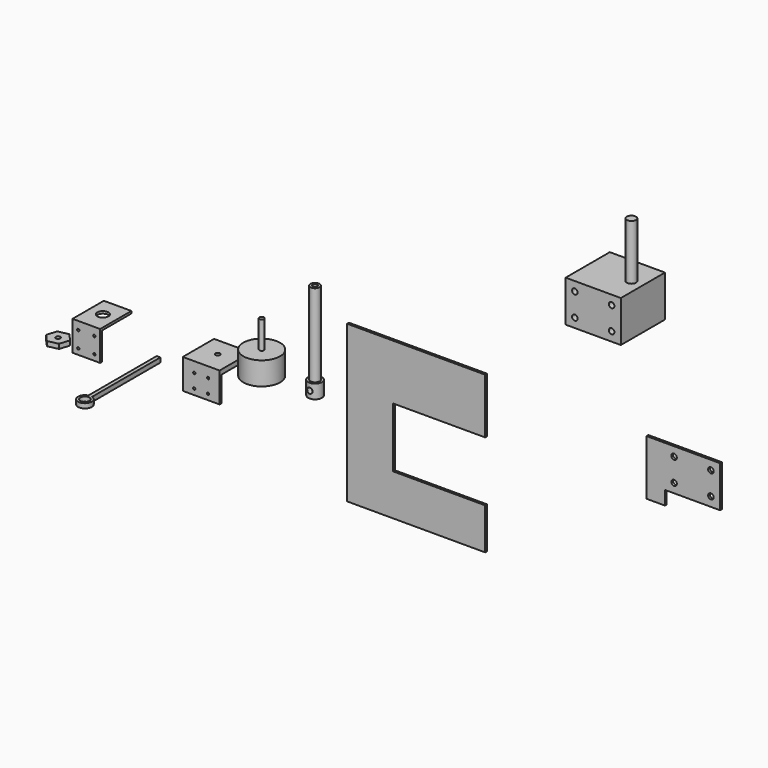
from build123d import *

# Parameters (mm, degrees)
F0_R      = 2.5
F1_DEPTH  = 15
F2_R      = 5
F2_R_2    = 2.5
F3_DEPTH  = 90
F5_R      = 3
F6_DEPTH  = 15.001
F0_R_2    = 20
F7_DEPTH  = 25
F8_R      = 2.5
F9_DEPTH  = 30
F0_W      = 40
F0_H      = 40
F10_DEPTH = 5
F11_W     = 40
F11_H     = 2.5
F12_DEPTH = 32.5
F14_DEPTH = 2.5
F0_W_2    = 30
F0_R_3    = 6
F16_DEPTH = 2.5
F17_W     = 30
F17_H     = 2.5
F18_DEPTH = 32.5
F19_DEPTH = 5
F20_R     = 1.25
F21_DEPTH = 2.5
F22_R     = 1.25
F23_DEPTH = 2.5
F13_W     = 60
F13_H     = 45
F13_R     = 3
F24_DEPTH = 60
F25_R     = 5
F26_DEPTH = 60
F27_DEPTH = 2.5
F28_R     = 3
F29_DEPTH = 25
F0_R_4    = 5
F30_DEPTH = 5


with BuildPart() as f1:
    # F0 (on Top) → F1 (new body)
    with BuildSketch(Plane.XY):
        with BuildLine():
            ThreePointArc((0, 7.5), (-5.3033008589, -5.3033008589), (7.5, 0))
            ThreePointArc((7.5, 0), (5.3033008589, 5.3033008589), (0, 7.5))
        make_face()
        Circle(F0_R, mode=Mode.SUBTRACT)
    extrude(amount=F1_DEPTH)

    # F2 (on face) → F3 (join)
    with BuildSketch(Plane.XY.offset(15)):
        Circle(F2_R)
        Circle(F2_R_2, mode=Mode.SUBTRACT)
    extrude(amount=F3_DEPTH)

    # F5 (on face) → F6 (cut, through all)
    with BuildSketch(Plane.XZ.offset(-7.5)):
        with Locations((0, 7.5)):
            Circle(F5_R)
    extrude(amount=F6_DEPTH, mode=Mode.SUBTRACT)


with BuildPart() as f7:
    # F0 (on Top) → F7 (new body)
    with BuildSketch(Plane.XY):
        with Locations((-57.9745993018, 0)):
            Circle(F0_R_2)
    extrude(amount=F7_DEPTH)

    # F8 (on face) → F9 (join)
    with BuildSketch(Plane.XY.offset(25)):
        with Locations((-57.9745993018, 0)):
            Circle(F8_R)
    extrude(amount=F9_DEPTH)


with BuildPart() as f10:
    # F0 (on Top) → F10 (new body)
    with BuildSketch(Plane.XY):
        with Locations((-105.7388707995, 0)):
            Rectangle(F0_W, F0_H)
        with Locations((-105.7388707995, 0)):
            Circle(F0_R, mode=Mode.SUBTRACT)
    extrude(amount=F10_DEPTH)

    # F11 (on face) → F12 (join)
    with BuildSketch(Plane.XY.offset(5)):
        with Locations((-105.7388707995, -21.25)):
            Rectangle(F11_W, F11_H)
    extrude(amount=-F12_DEPTH)

    # F20 (on face) → F21 (cut, through all)
    with BuildSketch(Plane(origin=(0, -20, 0), x_dir=(-1, 0, 0), z_dir=(0, 1, 0))):
        with Locations((98.2388707995, -6.25)):
            Circle(F20_R)
        with Locations((113.2388707995, -6.25)):
            Circle(F20_R)
        with Locations((113.2388707995, -21.25)):
            Circle(F20_R)
        with Locations((98.2388707995, -21.25)):
            Circle(F20_R)
    extrude(amount=-F21_DEPTH, mode=Mode.SUBTRACT)


with BuildPart() as f14:
    # F13 (on Front) → F14 (new body)
    with BuildSketch(Plane.XZ):
        Polygon((186.8768878281, 81.5050628316), (36.8768878281, 81.5050628316), (36.8768878281, -88.4949371684), (186.8768878281, -88.4949371684), (186.8768878281, -43.4949371684), (86.8768878281, -43.4949371684), (86.8768878281, 21.5050628316), (186.8768878281, 21.5050628316), align=None)
    extrude(amount=F14_DEPTH)


with BuildPart() as f16:
    # F0 (on Top) → F16 (new body)
    with BuildSketch(Plane.XY):
        with Locations((-230.5557584763, 0)):
            Rectangle(F0_W_2, F0_H)
        with Locations((-230.5557584763, 0)):
            Circle(F0_R_3, mode=Mode.SUBTRACT)
    extrude(amount=F16_DEPTH)

    # F17 (on face) → F18 (join)
    with BuildSketch(Plane.XY.offset(2.5)):
        with Locations((-230.5557584763, -21.25)):
            Rectangle(F17_W, F17_H)
    extrude(amount=-F18_DEPTH)

    # F22 (on face) → F23 (cut, through all)
    with BuildSketch(Plane(origin=(0, -20, 0), x_dir=(-1, 0, 0), z_dir=(0, 1, 0))):
        with Locations((221.8057584763, -6.25)):
            Circle(F22_R)
        with Locations((221.8057584763, -23.75)):
            Circle(F22_R)
        with Locations((239.3057584763, -23.75)):
            Circle(F22_R)
        with Locations((239.3057584763, -6.25)):
            Circle(F22_R)
    extrude(amount=-F23_DEPTH, mode=Mode.SUBTRACT)


with BuildPart() as f19:
    # F0 (on Top) → F19 (new body)
    with BuildSketch(Plane.XY):
        Polygon((-222.9001823011, -69.3075905842), (-219.3971571383, -58.4452201324), (-227.0527333135, -49.9803261255), (-238.2113346515, -52.3778025704), (-241.7143598142, -63.2401730222), (-234.058783639, -71.7050670291), align=None)
        with Locations((-230.5557584763, -60.8426965773)):
            Circle(F0_R, mode=Mode.SUBTRACT)
    extrude(amount=F19_DEPTH)


with BuildPart() as f24:
    # F13 (on Front) → F24 (new body)
    with BuildSketch(Plane.XZ):
        with Locations((302.3541259766, 178.6684757471)):
            Rectangle(F13_W, F13_H)
        with Locations((282.3541259766, 166.1684757471)):
            Circle(F13_R, mode=Mode.SUBTRACT)
        with Locations((282.3541259766, 191.1684757471)):
            Circle(F13_R, mode=Mode.SUBTRACT)
        with Locations((322.3541259766, 166.1684757471)):
            Circle(F13_R, mode=Mode.SUBTRACT)
        with Locations((322.3541259766, 191.1684757471)):
            Circle(F13_R, mode=Mode.SUBTRACT)
    extrude(amount=-F24_DEPTH)

    # F25 (on face) → F26 (join)
    with BuildSketch(Plane.XY.offset(201.1684757471)):
        with Locations((319.8541259766, 30)):
            Circle(F25_R)
    extrude(amount=F26_DEPTH)


with BuildPart() as f27:
    # F15 (on face) → F27 (new body)
    with BuildSketch(Plane.XZ.offset(2.5)):
        Polygon((444.2156124115, 81.5050628316), (364.2156124115, 81.5050628316), (364.2156124115, 21.5050628316), (384.2156124115, 21.5050628316), (384.2156124115, 36.5050628316), (444.2156124115, 36.5050628316), align=None)
    extrude(amount=F27_DEPTH)

    # F28 (on face) → F29 (cut)
    with BuildSketch(Plane.XZ.offset(5)):
        with Locations((394.2156124115, 71.5050628316)):
            Circle(F28_R)
        with Locations((394.2156124115, 46.5050628316)):
            Circle(F28_R)
        with Locations((434.2156124115, 71.5050628316)):
            Circle(F28_R)
        with Locations((434.2156124115, 46.5050628316)):
            Circle(F28_R)
    extrude(amount=-F29_DEPTH, mode=Mode.SUBTRACT)


with BuildPart() as f30:
    # F0 (on Top) → F30 (new body)
    with BuildSketch(Plane.XY):
        with BuildLine():
            Line((-144.055913806, -35.0423544645), (-144.055913806, -127.8139383171))
            ThreePointArc((-144.055913806, -127.8139383171), (-142.055913806, -142.5423544645), (-140.055913806, -127.8139383171))
            Line((-140.055913806, -127.8139383171), (-140.055913806, -35.0423544645))
            Line((-140.055913806, -35.0423544645), (-142.055913806, -35.0423544645))
            Line((-142.055913806, -35.0423544645), (-144.055913806, -35.0423544645))
        make_face()
        with Locations((-142.055913806, -135.0423544645)):
            Circle(F0_R_4, mode=Mode.SUBTRACT)
    extrude(amount=F30_DEPTH)


solid = Compound([f1.part, f7.part, f10.part, f14.part, f16.part, f19.part, f24.part, f27.part, f30.part])
